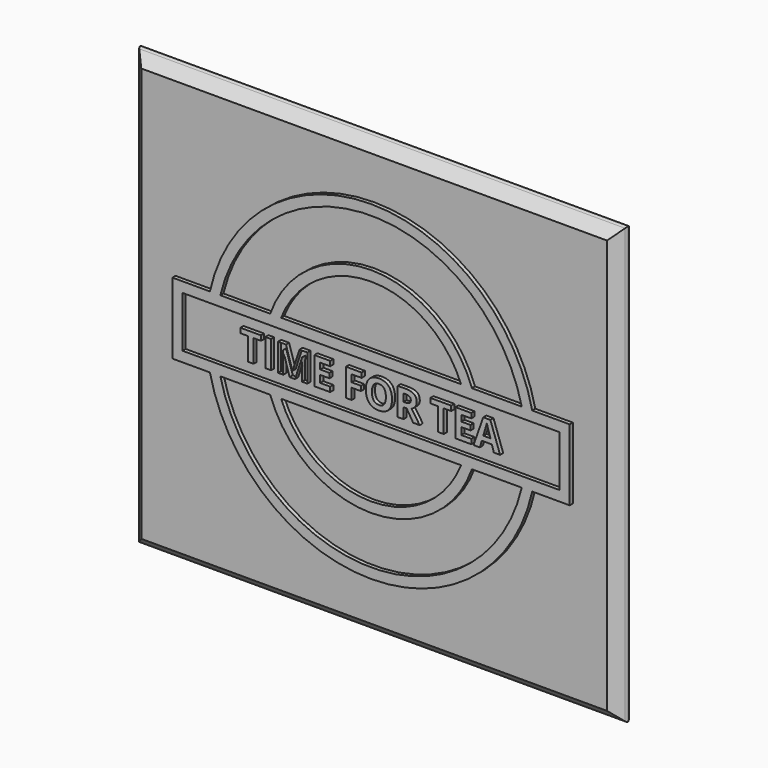
from build123d import *

# Parameters (mm, degrees)
F0_W         = 185
F0_H         = 25
F1_DEPTH     = 1.905
F2_W         = 247.65
F2_H         = 222.25
F3_DEPTH     = 7.62
F4_TEXT_SIZE = 18.8991388616
F5_DEPTH     = 1.905
F6_T1_DEPTH  = 271.2405609208
F6_T3_DEPTH  = 296.6405609208
F7_R         = 1.5875
F8_TEXT_SIZE = 29.9861111111
F9_DEPTH     = 0.762
F11_DEPTH    = 0.762


# Not quite as in the source:
# - a fillet or chamfer that OpenCascade refuses, or shapes differently, is made with other operations: its cross-section is extruded or revolved along the edge and cut away or added
# - Text() gives the source's letters only with a copy of the font that has no kerning and outlines rounded to 1/6400 em; it was checked with that copy


with BuildPart() as f1:
    # F0 (on Front) → F1 (new body)
    with BuildSketch(Plane.XZ):
        with BuildLine():
            Line((97.5, 17.5), (79.0869774362, 17.5))
            ThreePointArc((79.0869774362, 17.5), (0, 81), (-79.0869774362, 17.5))
            Line((-79.0869774362, 17.5), (-97.5, 17.5))
            Line((-97.5, 17.5), (-97.5, -17.5))
            Line((-97.5, -17.5), (-79.0869774362, -17.5))
            ThreePointArc((-79.0869774362, -17.5), (0, -81), (79.0869774362, -17.5))
            Line((79.0869774362, -17.5), (97.5, -17.5))
            Line((97.5, -17.5), (97.5, 17.5))
        make_face()
        with BuildLine():
            ThreePointArc((73.9577582137, -17.5), (0, -76), (-73.9577582137, -17.5))
            Line((-73.9577582137, -17.5), (-49.4974746831, -17.5))
            ThreePointArc((-49.4974746831, -17.5), (0, -52.5), (49.4974746831, -17.5))
            Line((49.4974746831, -17.5), (73.9577582137, -17.5))
        make_face(mode=Mode.SUBTRACT)
        with BuildLine():
            ThreePointArc((44.1588043316, -17.5), (0, -47.5), (-44.1588043316, -17.5))
            Line((-44.1588043316, -17.5), (44.1588043316, -17.5))
        make_face(mode=Mode.SUBTRACT)
        Rectangle(F0_W, F0_H, mode=Mode.SUBTRACT)
        with BuildLine():
            ThreePointArc((-44.1588043316, 17.5), (0, 47.5), (44.1588043316, 17.5))
            Line((44.1588043316, 17.5), (-44.1588043316, 17.5))
        make_face(mode=Mode.SUBTRACT)
        with BuildLine():
            ThreePointArc((-73.9577582137, 17.5), (0, 76), (73.9577582137, 17.5))
            Line((73.9577582137, 17.5), (49.4974746831, 17.5))
            ThreePointArc((49.4974746831, 17.5), (0, 52.5), (-49.4974746831, 17.5))
            Line((-49.4974746831, 17.5), (-73.9577582137, 17.5))
        make_face(mode=Mode.SUBTRACT)
    extrude(amount=F1_DEPTH)

    # F2 (on face) → F3 (join)
    with BuildSketch(Plane.XZ):
        Rectangle(F2_W, F2_H)
    extrude(amount=-F3_DEPTH)

    # F4 (on face) → F5 (join)
    with BuildSketch(Plane.XZ):
        with Locations((-64.5553241648, -6.8036899902)):
            Text('TIME FOR TEA', F4_TEXT_SIZE, font='Open Sans', font_style=FontStyle.BOLD, text_align=(TextAlign.LEFT, TextAlign.BOTTOM))
    extrude(amount=F5_DEPTH)

    # F6: chamfer of 9.525 on 4 edges, made by hand

    # F6_s2 → F6_t1 (cut)
    with BuildSketch(Plane.XY.offset(-135.6202804604)):
        Polygon((123.825, 9.525), (114.3, 0), (123.825, 0), align=None)
        Polygon((-114.3, 0), (-123.825, 9.525), (-123.825, 0), align=None)
    extrude(amount=F6_T1_DEPTH, mode=Mode.SUBTRACT)

    # F6_s4 → F6_t3 (cut)
    with BuildSketch(Plane.YZ.offset(-148.3202804604)):
        Polygon((9.525, 111.125), (0, 101.6), (0, 111.125), align=None)
        Polygon((9.525, -111.125), (0, -101.6), (0, -111.125), align=None)
    extrude(amount=F6_T3_DEPTH, mode=Mode.SUBTRACT)

    # F7
    f7_edges = [f1.edges().sort_by_distance(p)[0] for p in [
        (-121.92, 7.62, 0),
        (0, 7.62, 109.22),
        (121.92, 7.62, 0),
        (0, 7.62, -109.22),
    ]]
    fillet(f7_edges, radius=F7_R)

    # F8 (on face) → F9 (cut)
    with BuildSketch(Plane(origin=(0, 7.62, 0), x_dir=(-1, 0, 0), z_dir=(0, 1, 0))):
        with Locations(Location((83.0919824219, -20.955), (0, 0, 180))):
            Text('HAPPINESS', F8_TEXT_SIZE, font='Open Sans', font_style=FontStyle.BOLD, text_align=(TextAlign.LEFT, TextAlign.BOTTOM))
        with Locations(Location((82.110405816, 42.545), (0, 0, 180))):
            Text('TEA + CAKE', F8_TEXT_SIZE, font='Open Sans', font_style=FontStyle.BOLD, text_align=(TextAlign.LEFT, TextAlign.BOTTOM))
    extrude(amount=-F9_DEPTH, mode=Mode.SUBTRACT)

    # F10 (on face) → F11 (cut)
    with BuildSketch(Plane(origin=(0, 7.62, 0), x_dir=(-1, 0, 0), z_dir=(0, 1, 0))):
        with BuildLine():
            Line((105.6005, 100.0125), (-105.6005, 100.0125))
            ThreePointArc((-105.6005, 100.0125), (-110.6294434278, 97.9294434278), (-112.7125, 92.9005))
            Line((-112.7125, 92.9005), (-112.7125, -92.9005))
            ThreePointArc((-112.7125, -92.9005), (-110.6294434278, -97.9294434278), (-105.6005, -100.0125))
            Line((-105.6005, -100.0125), (105.6005, -100.0125))
            ThreePointArc((105.6005, -100.0125), (110.6294434278, -97.9294434278), (112.7125, -92.9005))
            Line((112.7125, -92.9005), (112.7125, 92.9005))
            ThreePointArc((112.7125, 92.9005), (110.6294434278, 97.9294434278), (105.6005, 100.0125))
        make_face()
        with BuildLine():
            ThreePointArc((-108.9025, 93.6625), (-108.1585512242, 95.4585512242), (-106.3625, 96.2025))
            Line((-106.3625, 96.2025), (106.3625, 96.2025))
            ThreePointArc((106.3625, 96.2025), (108.1585512242, 95.4585512242), (108.9025, 93.6625))
            Line((108.9025, 93.6625), (108.9025, -93.6625))
            ThreePointArc((108.9025, -93.6625), (108.1585512242, -95.4585512242), (106.3625, -96.2025))
            Line((106.3625, -96.2025), (-105.6005, -96.2025))
            ThreePointArc((-105.6005, -96.2025), (-107.9353665915, -95.2353665915), (-108.9025, -92.9005))
            Line((-108.9025, -92.9005), (-108.9025, 93.6625))
        make_face(mode=Mode.SUBTRACT)
        with BuildLine():
            Line((105.6005, 94.4245), (-105.6005, 94.4245))
            ThreePointArc((-105.6005, 94.4245), (-106.6781307345, 93.9781307345), (-107.1245, 92.9005))
            Line((-107.1245, 92.9005), (-107.1245, -92.9005))
            ThreePointArc((-107.1245, -92.9005), (-106.6781307345, -93.9781307345), (-105.6005, -94.4245))
            Line((-105.6005, -94.4245), (105.6005, -94.4245))
            ThreePointArc((105.6005, -94.4245), (106.6781307345, -93.9781307345), (107.1245, -92.9005))
            Line((107.1245, -92.9005), (107.1245, 92.9005))
            ThreePointArc((107.1245, 92.9005), (106.6781307345, 93.9781307345), (105.6005, 94.4245))
        make_face()
        with BuildLine():
            ThreePointArc((-106.1085, 92.9005), (-105.9597102448, 93.2597102448), (-105.6005, 93.4085))
            Line((-105.6005, 93.4085), (105.6005, 93.4085))
            ThreePointArc((105.6005, 93.4085), (105.9597102448, 93.2597102448), (106.1085, 92.9005))
            Line((106.1085, 92.9005), (106.1085, -92.9005))
            ThreePointArc((106.1085, -92.9005), (105.9597102448, -93.2597102448), (105.6005, -93.4085))
            Line((105.6005, -93.4085), (-105.6005, -93.4085))
            ThreePointArc((-105.6005, -93.4085), (-105.9597102448, -93.2597102448), (-106.1085, -92.9005))
            Line((-106.1085, -92.9005), (-106.1085, 92.9005))
        make_face(mode=Mode.SUBTRACT)
    extrude(amount=-F11_DEPTH, mode=Mode.SUBTRACT)


solid = f1.part
